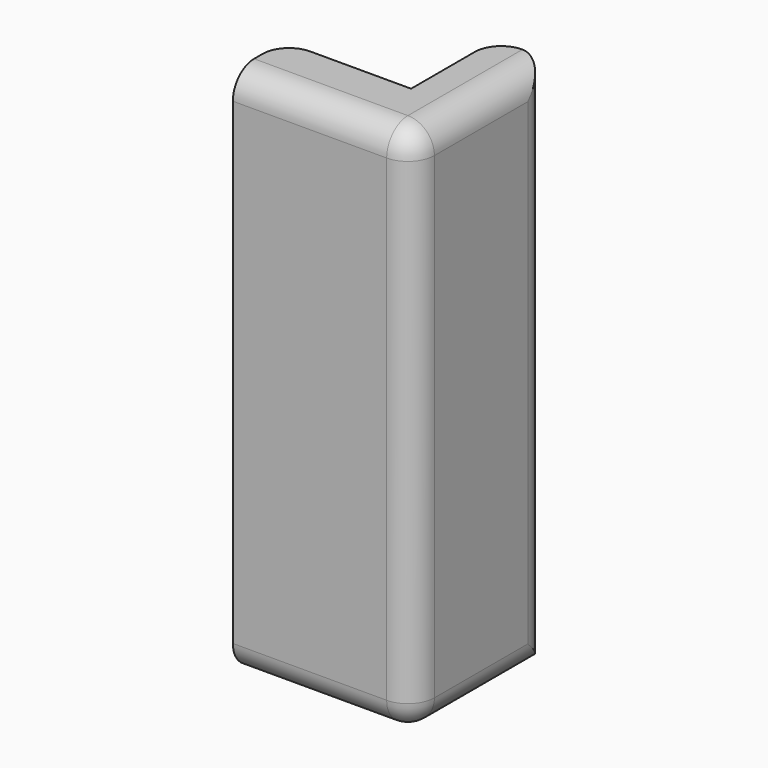
from build123d import *

# Parameters (mm, degrees)
F1_DEPTH      = 50
F1_DEPTH_BACK = 50
F2_W          = 10
F2_H          = 45
F3_DEPTH      = 5
F4_R          = 6
F5_DEPTH      = 3
F6_R          = 4.99999


# Not quite as in the source:
# - a fillet or chamfer is up to 0.001 mm smaller than in the source, because OpenCascade refuses the exact size


with BuildPart() as f1:
    # F0 (on Top) → F1 (new body, two sides)
    with BuildSketch(Plane.XY) as f1_sk:
        Polygon((0, -12), (0, 0), (0, 20), (-10, 20), (-10, 0), (-34, 0), (-34, -12), align=None)
    extrude(amount=F1_DEPTH)
    extrude(f1_sk.sketch, amount=-F1_DEPTH_BACK)

    # F2 (on face) → F3 (join)
    with BuildSketch(Plane(origin=(0, 0, 0), x_dir=(-1, 0, 0), z_dir=(0, 1, 0))):
        with Locations((19, 5.5)):
            Rectangle(F2_W, F2_H)
    extrude(amount=F3_DEPTH)

    # F4 (on face) → F5 (cut)
    with BuildSketch(Plane(origin=(0, 0, 0), x_dir=(-1, 0, 0), z_dir=(0, 1, 0))):
        with Locations((22, 39)):
            Circle(F4_R)
        with Locations((22, -33.5)):
            Circle(F4_R)
    extrude(amount=-F5_DEPTH, mode=Mode.SUBTRACT)

    # F6 (radius 5 in the source; OpenCascade refuses exactly that, so slightly less here)
    f6_edges = [f1.edges().sort_by_distance(p)[0] for p in [
        (0, -12, 0),
        (0, 4, 50),
        (-17, -12, 50),
        (-17, -12, -50),
        (0, 4, -50),
        (-10, 20, 0),
        (0, 20, 0),
        (-34, 0, 0),
    ]]
    fillet(f6_edges, radius=F6_R)


solid = f1.part
